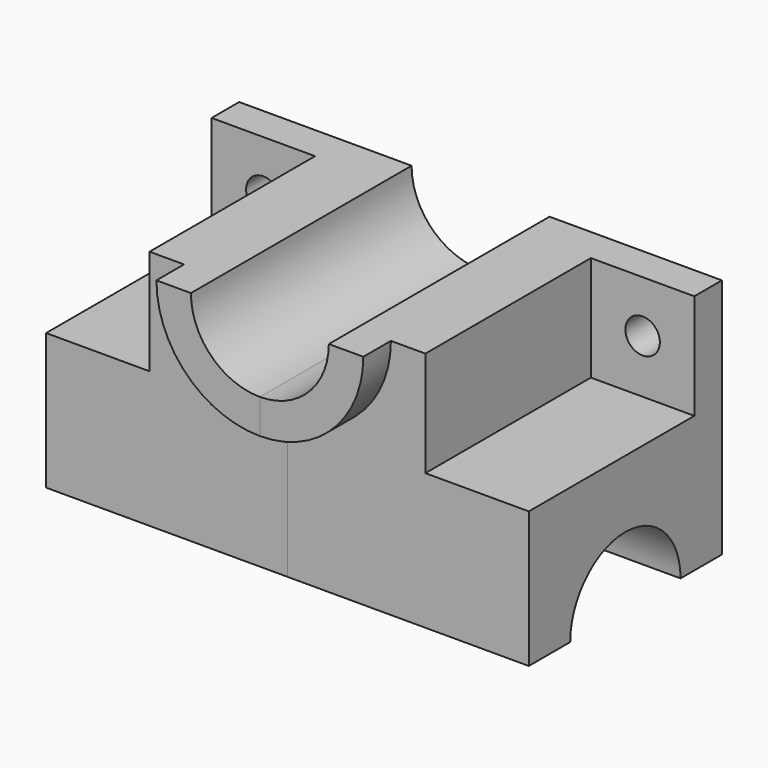
from build123d import *
from build123d import SkipClean  # not in build123d's __all__

# Parameters (mm, degrees)
F1_DEPTH = 70
F2_W     = 30
F2_H     = 30.5260747812
F3_DEPTH = 60
F4_R     = 5
F5_DEPTH = 10.001
F6_R     = 20
F7_DEPTH = 70.001
F9_DEPTH = 10


with BuildPart() as f1:
    # F0 (on Front) → F1 (new body)
    with BuildSketch(Plane.XZ):
        with BuildLine():
            Line((0, -20), (0, -70))
            Line((0, -70), (70, -70))
            Line((70, -70), (70, 0))
            Line((70, 0), (20, 0))
            ThreePointArc((20, 0), (14.1421356237, -14.1421356237), (0, -20))
        make_face()
    extrude(amount=-F1_DEPTH)

    # F2 (on face) → F3 (cut)
    with BuildSketch(Plane.XZ):
        with Locations((55, -15.2630373906)):
            Rectangle(F2_W, F2_H)
    extrude(amount=-F3_DEPTH, mode=Mode.SUBTRACT)

    # F4 (on face) → F5 (cut, through all)
    with BuildSketch(Plane.XZ.offset(-60)):
        with Locations((55, -15)):
            Circle(F4_R)
    extrude(amount=-F5_DEPTH, mode=Mode.SUBTRACT)

    # F6 (on face) → F7 (cut, through all)
    with BuildSketch(Plane.YZ.offset(70)):
        with Locations((35, -70)):
            Circle(F6_R)
    extrude(amount=-F7_DEPTH, mode=Mode.SUBTRACT)

    # F8 (on face) → F9 (join)
    with BuildSketch(Plane.XZ):
        with BuildLine():
            ThreePointArc((20, 0), (14.1421356237, -14.1421356237), (0, -20))
            Line((0, -20), (0, -30))
            ThreePointArc((0, -30), (21.2132034356, -21.2132034356), (30, 0))
            Line((30, 0), (20, 0))
        make_face()
    extrude(amount=F9_DEPTH)

    # F10: F1 across plane


with BuildPart() as f1_1:
    add(f1.part, clean=False)
    with SkipClean():  # cleaning this boolean's faces spoils the solid; the shape is the same uncleaned
        add(f1.part.mirror(Plane.YZ), clean=False)


solid = f1_1.part
